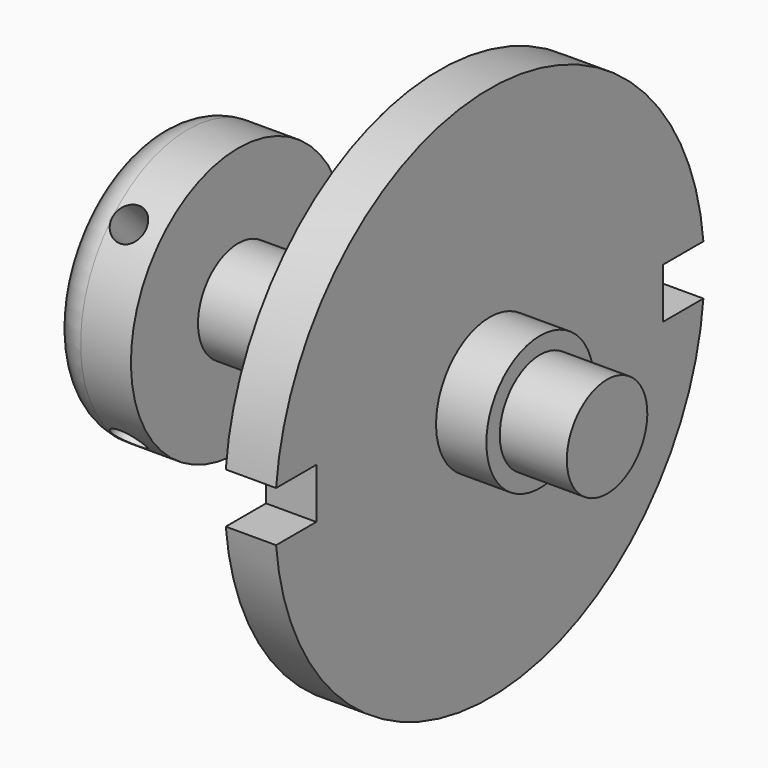
from build123d import *

# Parameters (mm, degrees)
F2_R             = 9.525
F3_DEPTH         = 20.828
F4_SIZE          = 5.08
F5_R             = 9.525
F6_DEPTH         = 20.828
F7_SIZE          = 5.08
F9_DEPTH         = 25.4
F11_DEPTH        = 25.4
F14_R            = 6.35
F15_DEPTH        = 25.4
F15_COPIES_COUNT = 4


# Not quite as in the source:
# - a pattern or mirror of a feature is missing from the dataset's text; its kind, count and spacing are read off the source's solid


with BuildPart() as f1:
    # F0 (on Front) → F1 (revolve)
    with BuildSketch(Plane.XZ):
        with BuildLine():
            Line((-171.45, 0), (0, 0))
            Line((0, 0), (0, 19.05))
            Line((0, 19.05), (-25.4, 19.05))
            Line((-25.4, 19.05), (-25.4, 25.4))
            Line((-25.4, 25.4), (-44.45, 25.4))
            Line((-44.45, 25.4), (-44.45, 101.6))
            Line((-44.45, 101.6), (-63.5, 101.6))
            Line((-63.5, 101.6), (-63.5, 19.05))
            Line((-63.5, 19.05), (-139.7, 19.05))
            Line((-139.7, 19.05), (-139.7, 50.8))
            Line((-139.7, 50.8), (-158.75, 50.8))
            ThreePointArc((-158.75, 50.8), (-167.7302561211, 47.0802561211), (-171.45, 38.1))
            Line((-171.45, 38.1), (-171.45, 0))
        make_face()
    revolve(axis=Axis((-33.1432974098, 0, 0), (1, 0, 0)))

    # F2 (on face) → F3 (join)
    with BuildSketch(Plane(origin=(-63.5, 0, 0), x_dir=(0, -1, 0), z_dir=(-1, 0, 0))):
        with Locations((0, 76.2)):
            Circle(F2_R)
    extrude(amount=F3_DEPTH)

    # F4
    f4_edges = [f1.edges().sort_by_distance(p)[0] for p in [
        (-84.328, 9.525, 76.2),
    ]]
    chamfer(f4_edges, length=F4_SIZE)

    # F8 (on face) → F9 (cut)
    with BuildSketch(Plane(origin=(-63.5, 0, 0), x_dir=(0, -1, 0), z_dir=(-1, 0, 0))):
        with BuildLine():
            Line((-82.1025302452, 9.525), (-101.1525302452, 9.525))
            ThreePointArc((-101.1525302452, 9.525), (-101.6, 0), (-101.1525302452, -9.525))
            Line((-101.1525302452, -9.525), (-82.1025302452, -9.525))
            Line((-82.1025302452, -9.525), (-82.1025302452, 9.525))
        make_face()
    extrude(amount=-F9_DEPTH, mode=Mode.SUBTRACT)

    # F10 (on face) → F11 (cut)
    with BuildSketch(Plane(origin=(-63.5, 0, 0), x_dir=(0, -1, 0), z_dir=(-1, 0, 0))):
        with BuildLine():
            ThreePointArc((101.1525302452, -9.525), (101.6, 0), (101.1525302452, 9.525))
            Line((101.1525302452, 9.525), (82.1025302452, 9.525))
            Line((82.1025302452, 9.525), (82.1025302452, -9.525))
            Line((82.1025302452, -9.525), (101.1525302452, -9.525))
        make_face()
    extrude(amount=-F11_DEPTH, mode=Mode.SUBTRACT)

    # F14 (on line) → F15 (cut)
    with BuildSketch(Plane(origin=(0, -35.9210244843, 35.9210244843), x_dir=(1, 0, 0), z_dir=(0, -0.7071067812, 0.7071067812))):
        with Locations((-152.4, 0)):
            Circle(F14_R)
    f15 = extrude(amount=-F15_DEPTH, mode=Mode.SUBTRACT)

    # F15_copies: F15 ×4 about axis
    f15_copies_axis = Axis((0, 0, 0), (1, 0, 0))
    for i in range(1, F15_COPIES_COUNT):
        add(f15.rotate(f15_copies_axis, i * 360 / F15_COPIES_COUNT), mode=Mode.SUBTRACT)


with BuildPart() as f6:
    # F5 (on face) → F6 (new body)
    with BuildSketch(Plane(origin=(-63.5, 0, 0), x_dir=(0, -1, 0), z_dir=(-1, 0, 0))):
        with Locations((0, -76.2)):
            Circle(F5_R)
    extrude(amount=F6_DEPTH)

    # F7
    f7_edges = [f6.edges().sort_by_distance(p)[0] for p in [
        (-84.328, 9.525, -76.2),
    ]]
    chamfer(f7_edges, length=F7_SIZE)


solid = Compound([f1.part, f6.part])
